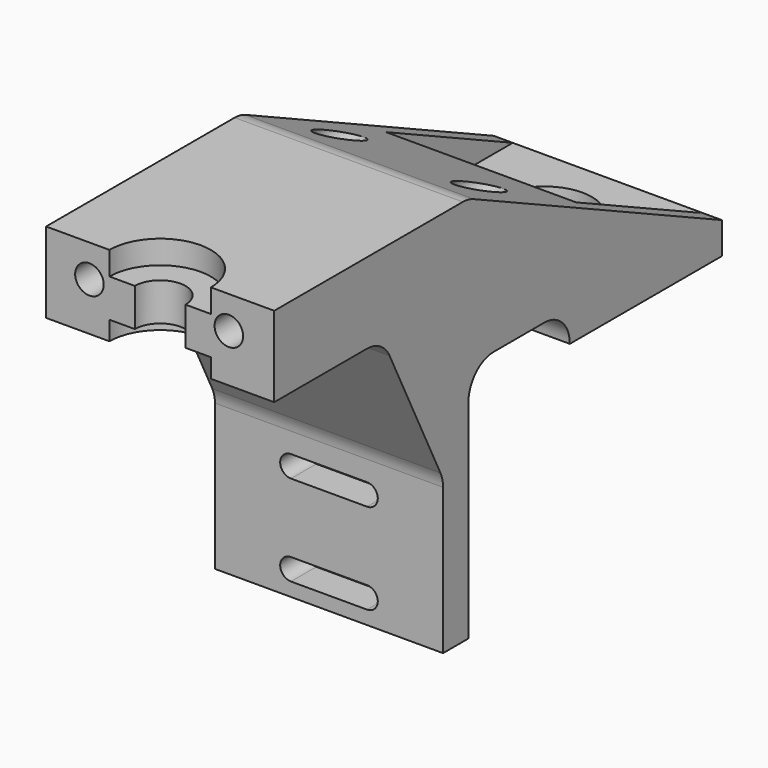
from build123d import *

# Parameters (mm, degrees)
F0_W      = 30
F0_H      = 22
F1_DEPTH  = 5
F2_DEPTH  = 39.1
F3_W      = 30
F3_H      = 12.7
F4_DEPTH  = 50
F8_W      = 30
F8_H      = 5
F9_DEPTH  = 25
F10_W     = 30
F10_H     = 5
F11_DEPTH = 5
F12_W     = 30
F12_H     = 5
F13_DEPTH = 25
F15_DEPTH = 25
F16_DEPTH = 3
F18_DEPTH = 3
F19_DEPTH = 3
F21_DEPTH = 3
F23_DEPTH = 30
F24_R     = 2.25
F25_DEPTH = 500
F26_W     = 68.0921077728
F26_H     = 72.8289508261
F27_DEPTH = 25
F29_DEPTH = 36
F30_R     = 4.99999
F32_DEPTH = 1


# Not quite as in the source:
# - a fillet or chamfer is up to 0.001 mm smaller than in the source, because OpenCascade refuses the exact size


with BuildPart() as f1:
    # F0 (on Front) → F1 (new body)
    with BuildSketch(Plane.XZ):
        with Locations((0, 7.15)):
            Rectangle(F0_W, F0_H)
        with BuildLine():
            ThreePointArc((-6, -1.7), (-7.7, 0), (-6, 1.7))
            Line((-6, 1.7), (6, 1.7))
            ThreePointArc((6, 1.7), (7.7, 0), (6, -1.7))
            Line((6, -1.7), (-6, -1.7))
        make_face(mode=Mode.SUBTRACT)
        with BuildLine():
            ThreePointArc((-6, 12.6), (-7.7, 14.3), (-6, 16))
            Line((-6, 16), (6, 16))
            ThreePointArc((6, 16), (7.7, 14.3), (6, 12.6))
            Line((6, 12.6), (-6, 12.6))
        make_face(mode=Mode.SUBTRACT)
    extrude(amount=F1_DEPTH)

    # F2 (add): a face of the model
    f2_faces = [f1.faces().sort_by_distance(p)[0] for p in [
        (0, -2.5, 18.15),
    ]]
    extrude(f2_faces, amount=F2_DEPTH)

    # F3 (on face) → F4 (join)
    with BuildSketch(Plane.XZ.offset(5)):
        with Locations((0, 50.9)):
            Rectangle(F3_W, F3_H)
    extrude(amount=F4_DEPTH)

    # F6 (on offset) → F7 (revolve, cut)
    with BuildSketch(Plane.XZ.offset(38.3)):
        Polygon((8, 57.25), (0, 57.25), (0, 44.55), (8, 44.55), (8, 47.55), (4, 47.55), (4, 53.55), (8, 53.55), align=None)
    revolve(axis=Axis((0, -38.3, 50.9), (0, 0, 1)), mode=Mode.SUBTRACT)

    # F8 (on face) → F9 (join)
    with BuildSketch(Plane(origin=(0, 0, 0), x_dir=(-1, 0, 0), z_dir=(0, 1, 0))):
        with Locations((0, 36.45)):
            Rectangle(F8_W, F8_H)
    extrude(amount=F9_DEPTH)

    # F10 (on face) → F11 (join)
    with BuildSketch(Plane(origin=(0, 0, 33.95), x_dir=(1, 0, 0), z_dir=(0, 0, -1))):
        with Locations((0, -22.5)):
            Rectangle(F10_W, F10_H)
    extrude(amount=F11_DEPTH)

    # F12 (on face) → F13 (join)
    with BuildSketch(Plane(origin=(0, 25, 0), x_dir=(-1, 0, 0), z_dir=(0, 1, 0))):
        with Locations((0, 31.45)):
            Rectangle(F12_W, F12_H)
    extrude(amount=F13_DEPTH)

    # F14 (on face) → F15 (cut)
    with BuildSketch(Plane.XY.offset(33.95)):
        with BuildLine():
            ThreePointArc((7.4548611111, 38.3216117173), (0, 45), (-7.4548611111, 38.3216117173))
            ThreePointArc((-7.4548611111, 38.3216117173), (-10.75, 37.5), (-7.4548611111, 36.6783882827))
            ThreePointArc((-7.4548611111, 36.6783882827), (0, 30), (7.4548611111, 36.6783882827))
            ThreePointArc((7.4548611111, 36.6783882827), (10.75, 37.5), (7.4548611111, 38.3216117173))
        make_face()
    extrude(amount=-F15_DEPTH, mode=Mode.SUBTRACT)

    # F16 (add): a face of the model
    f16_faces = [f1.faces().sort_by_distance(p)[0] for p in [
        (15, -2.5, -2.6351662665),
    ]]
    extrude(f16_faces, amount=F16_DEPTH)

    # F17 (on face) → F18 (join)
    with BuildSketch(Plane.YZ.offset(18)):
        Polygon((50, 33.95), (0, 57.25), (0, 38.95), (25, 38.95), (25, 33.95), align=None)
    extrude(amount=-F18_DEPTH)

    # F19 (add): a face of the model
    f19_faces = [f1.faces().sort_by_distance(p)[0] for p in [
        (-15, -2.5, -2.6351662665),
    ]]
    extrude(f19_faces, amount=F19_DEPTH)

    # F20 (on face) → F21 (join)
    with BuildSketch(Plane(origin=(-18, 0, 0), x_dir=(0, -1, 0), z_dir=(-1, 0, 0))):
        Polygon((0, 57.25), (-50, 33.95), (-25, 33.95), (-25, 38.95), (0, 38.95), align=None)
    extrude(amount=-F21_DEPTH)

    # F22 (on face) → F23 (join, through all)
    with BuildSketch(Plane(origin=(15, 0, 0), x_dir=(0, -1, 0), z_dir=(-1, 0, 0))):
        Polygon((-25, 45.6), (-25, 38.95), (0, 38.95), (0, 57.25), align=None)
    extrude(amount=F23_DEPTH)

    # F24 (on face) → F25 (cut)
    with BuildSketch(Plane.XZ.offset(55)):
        with Locations((-11.1628601777, 52.1221570671)):
            Circle(F24_R)
        with Locations((10.8371398223, 52.1221570671)):
            Circle(F24_R)
    extrude(amount=-F25_DEPTH, mode=Mode.SUBTRACT)

    # F26 (on offset) → F27 (cut)
    with BuildSketch(Plane.XZ.offset(38.3)):
        with Locations((0.2960525453, 29.3092119973)):
            Rectangle(F26_W, F26_H)
    extrude(amount=F27_DEPTH, mode=Mode.SUBTRACT)

    # F28 (on face) → F29 (join)
    with BuildSketch(Plane(origin=(-18, 0, 0), x_dir=(0, -1, 0), z_dir=(-1, 0, 0))):
        Polygon((5, 44.55), (5, 20.35), (16.9268529862, 44.55), align=None)
    extrude(amount=-F29_DEPTH)

    # F30 (radius 5 in the source; OpenCascade refuses exactly that, so slightly less here)
    f30_edges = [f1.edges().sort_by_distance(p)[0] for p in [
        (0, -16.926853, 44.55),
        (0, 0, 57.25),
        (0, 20, 33.95),
        (0, 0, 33.95),
        (0, -5, 20.35),
    ]]
    fillet(f30_edges, radius=F30_R)

    # F31 (on face) → F32 (cut)
    with BuildSketch(Plane(origin=(-18, 0, 0), x_dir=(0, -1, 0), z_dir=(-1, 0, 0))):
        with BuildLine():
            ThreePointArc((-2.9166666459, 43.103029569), (-2.2332491353, 41.4531137462), (-0.5833333125, 40.7696962357))
            Line((-0.5833333125, 40.7696962357), (6.4166666875, 40.7696962357))
            ThreePointArc((6.4166666875, 40.7696962357), (8.0665825102, 41.4531137462), (8.7500000208, 43.103029569))
            Line((8.7500000208, 43.103029569), (8.7500000208, 50.103029569))
            ThreePointArc((8.7500000208, 50.103029569), (8.0665825102, 51.7529453918), (6.4166666875, 52.4363629023))
            Line((6.4166666875, 52.4363629023), (-0.5833333125, 52.4363629023))
            ThreePointArc((-0.5833333125, 52.4363629023), (-2.2332491353, 51.7529453918), (-2.9166666459, 50.103029569))
            Line((-2.9166666459, 50.103029569), (-2.9166666459, 43.103029569))
        make_face()
        with BuildLine():
            Line((4.6666666875, 43.103029569), (1.1666666875, 43.103029569))
            ThreePointArc((1.1666666875, 43.103029569), (-0.0707701796, 43.6155927019), (-0.5833333125, 44.853029569))
            Line((-0.5833333125, 44.853029569), (-0.5833333125, 48.353029569))
            ThreePointArc((-0.5833333125, 48.353029569), (-0.0707701796, 49.5904664361), (1.1666666875, 50.103029569))
            Line((1.1666666875, 50.103029569), (4.6666666875, 50.103029569))
            ThreePointArc((4.6666666875, 50.103029569), (5.9041035545, 49.5904664361), (6.4166666875, 48.353029569))
            Line((6.4166666875, 48.353029569), (6.4166666875, 44.853029569))
            ThreePointArc((6.4166666875, 44.853029569), (6.3861771815, 44.5277855668), (6.2957710749, 44.2138747406))
            Line((6.2957710875, 44.2138747357), (3.8241204375, 46.6855253857))
            ThreePointArc((3.8241204265, 46.6855253747), (3.4116414708, 46.8563797523), (2.9991625151, 46.6855253747))
            Line((2.9991625041, 46.6855253857), (2.9166666875, 46.603029569))
            Line((2.9166666875, 46.603029569), (2.8341708708, 46.5205337523))
            ThreePointArc((2.8341708818, 46.5205337413), (2.6633165041, 46.1080547857), (2.8341708818, 45.69557583))
            Line((2.8341708708, 45.695575819), (5.3058215208, 43.223925169))
            ThreePointArc((5.3058215159, 43.2239251815), (4.9919106896, 43.133519075), (4.6666666875, 43.103029569))
        make_face(mode=Mode.SUBTRACT)
    extrude(amount=-F32_DEPTH, mode=Mode.SUBTRACT)


solid = f1.part
